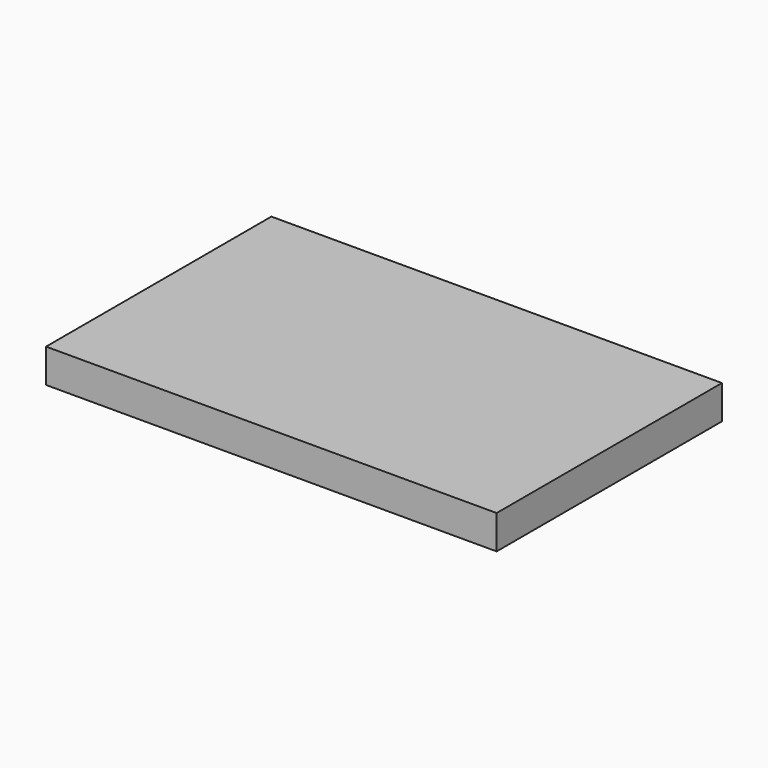
from build123d import *

# Parameters (mm, degrees)
F0_W     = 40
F0_H     = 25
F2_DEPTH = 1.5
F3_W     = 40
F3_H     = 25
F3_W_2   = 36
F3_H_2   = 21
F4_DEPTH = 1.5


# Not quite as in the source:
# - the program builds the solid bodies; features that only make, move or delete a surface that nothing else refers to are left out


with BuildPart() as f2:
    # F0 (on Top) → F2 (new body)
    with BuildSketch(Plane.XY):
        Rectangle(F0_W, F0_H)
    extrude(amount=F2_DEPTH)

    # F3 (on face) → F4 (join)
    with BuildSketch(Plane(origin=(0, 0, 0), x_dir=(1, 0, 0), z_dir=(0, 0, -1))):
        Rectangle(F3_W, F3_H)
        Rectangle(F3_W_2, F3_H_2, mode=Mode.SUBTRACT)
    extrude(amount=F4_DEPTH)


solid = f2.part
